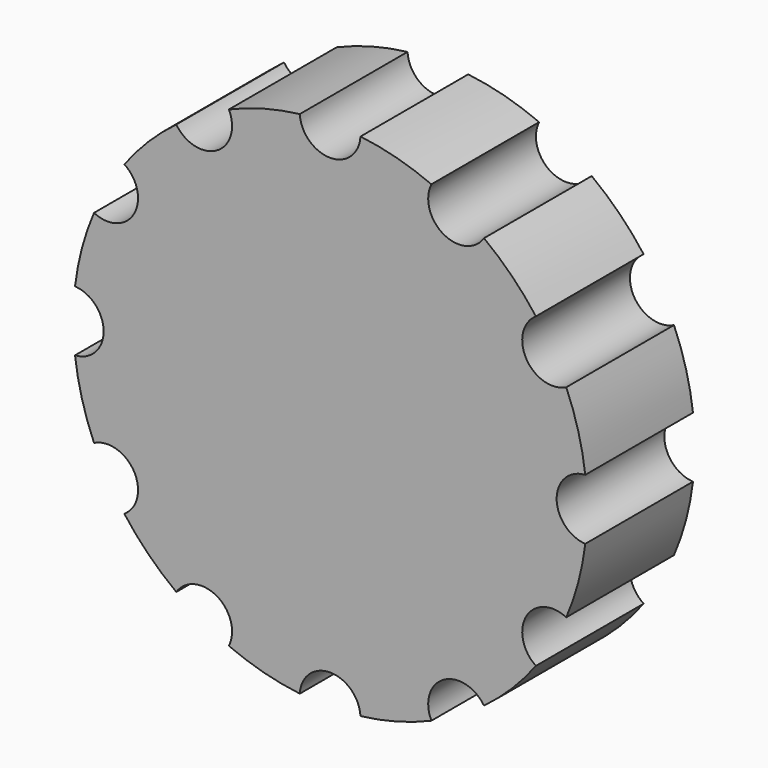
from build123d import *

# Parameters (mm, degrees)
F0_R            = 47.6973653994
F1_DEPTH        = 25
F3_DEPTH        = 25
F3_COPIES_COUNT = 12


# Not quite as in the source:
# - a feature of the source that left no trace in its solid (it failed there, or was rolled back) is left out
# - a pattern or mirror of a feature is missing from the dataset's text; its kind, count and spacing are read off the source's solid


with BuildPart() as f1:
    # F0 (on Front) → F1 (new body)
    with BuildSketch(Plane.XZ):
        Circle(F0_R)
    extrude(amount=F1_DEPTH)

    # F2 (on face) → F3 (cut)
    with BuildSketch(Plane.XZ.offset(25)):
        with BuildLine():
            ThreePointArc((5.635130152, 47.3633188683), (0, 47.6973653994), (-5.635130152, 47.3633188683))
            ThreePointArc((-5.635130152, 47.3633188683), (0, 42.0523429092), (5.635130152, 47.3633188683))
        make_face()
    f3 = extrude(amount=-F3_DEPTH, mode=Mode.SUBTRACT)

    # F3_copies: F3 ×12 about axis
    f3_copies_axis = Axis((0, 0, 0), (0, 1, 0))
    for i in range(1, F3_COPIES_COUNT):
        add(f3.rotate(f3_copies_axis, i * 360 / F3_COPIES_COUNT), mode=Mode.SUBTRACT)


solid = f1.part
